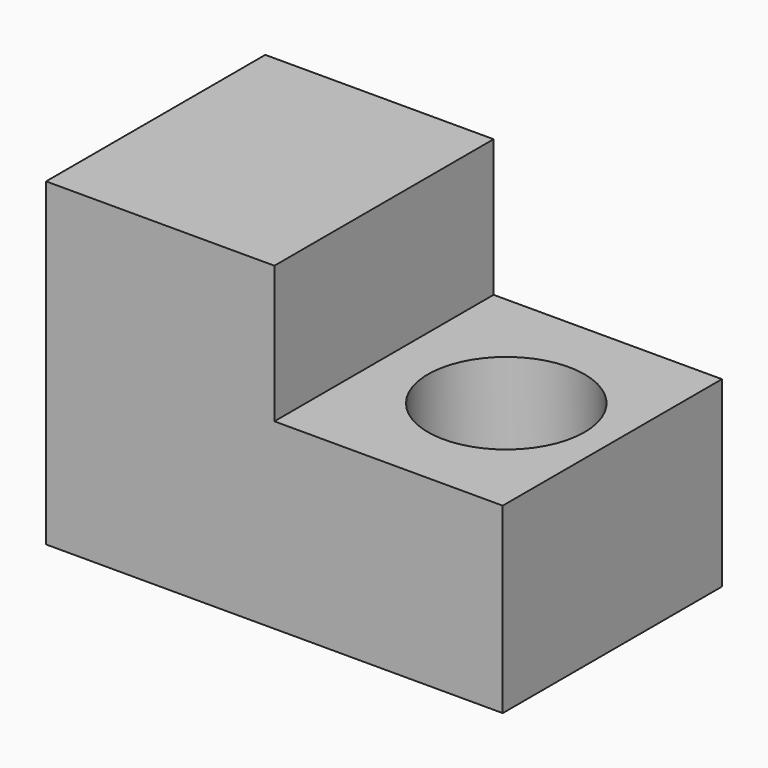
from build123d import *

# Parameters (mm, degrees)
F1_DEPTH = 762
F2_R     = 217.8858008063
F3_DEPTH = 508


# Not quite as in the source:
# - a feature names something its author has since deleted; it is built from what else it names


with BuildPart() as f1:
    # F0 (on Front) → F1 (new body)
    with BuildSketch(Plane.XZ):
        Polygon((-1270, 0), (0, 0), (0, 508), (-635, 508), (-635, 889), (-1270, 889), align=None)
    extrude(amount=F1_DEPTH)

    # F2 (on face) → F3 (cut)
    with BuildSketch(Plane.XY.offset(508)):
        with Locations((-295.0017750263, -381)):
            Circle(F2_R)
    extrude(amount=-F3_DEPTH, mode=Mode.SUBTRACT)


solid = f1.part
